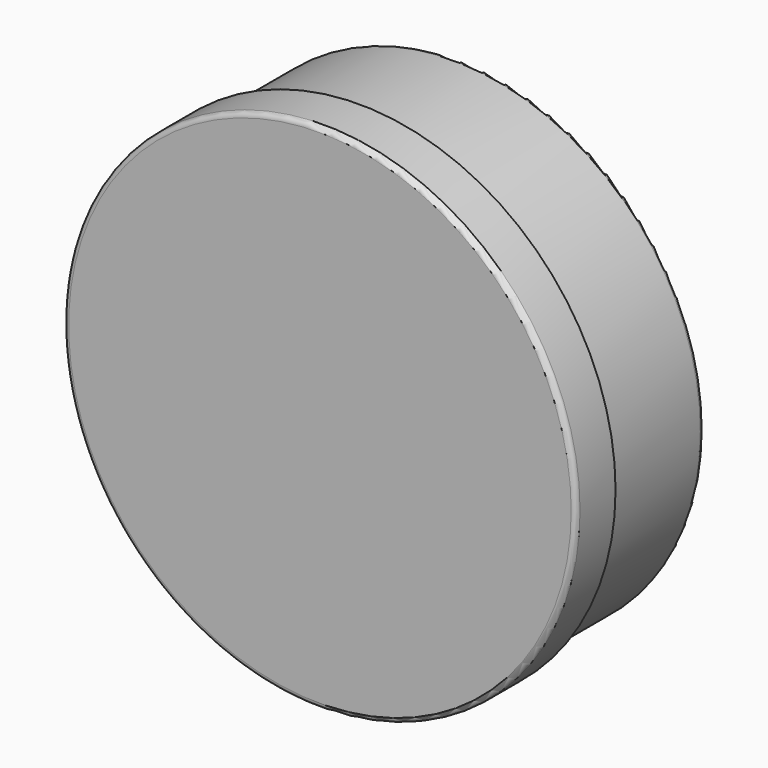
from build123d import *

# Parameters (mm, degrees)
F0_R     = 50
F1_DEPTH = 25
F2_R     = 52
F2_R_2   = 50
F3_DEPTH = 10
F5_T     = -1.5
F6_R     = 33.5
F6_R_2   = 31.5
F7_DEPTH = 5
F8_R     = 1


# Not quite as in the source:
# - a feature of the source that left no trace in its solid (it failed there, or was rolled back) is left out


with BuildPart() as f1:
    # F0 (on Front) → F1 (new body)
    with BuildSketch(Plane.XZ):
        Circle(F0_R)
    extrude(amount=F1_DEPTH)

    # F2 (on face) → F3 (join)
    with BuildSketch(Plane.XZ.offset(25)):
        Circle(F2_R)
        Circle(F2_R_2, mode=Mode.SUBTRACT)
        Circle(F2_R_2)
    extrude(amount=F3_DEPTH)

    # F5
    f5_openings = [f1.faces().sort_by_distance(p)[0] for p in [
        (0, 0, 0),
    ]]
    offset(amount=F5_T, openings=f5_openings, kind=Kind.INTERSECTION)

    # F6 (on face) → F7 (join)
    with BuildSketch(Plane(origin=(0, -33.5, 0), x_dir=(-1, 0, 0), z_dir=(0, 1, 0))):
        Circle(F6_R)
        Circle(F6_R_2, mode=Mode.SUBTRACT)
    extrude(amount=F7_DEPTH)

    # F8
    f8_edges = [f1.edges().sort_by_distance(p)[0] for p in [
        (31.5, -28.5, 0),
        (-52, -35, 0),
        (-50, 0, 0),
    ]]
    fillet(f8_edges, radius=F8_R)


solid = f1.part
